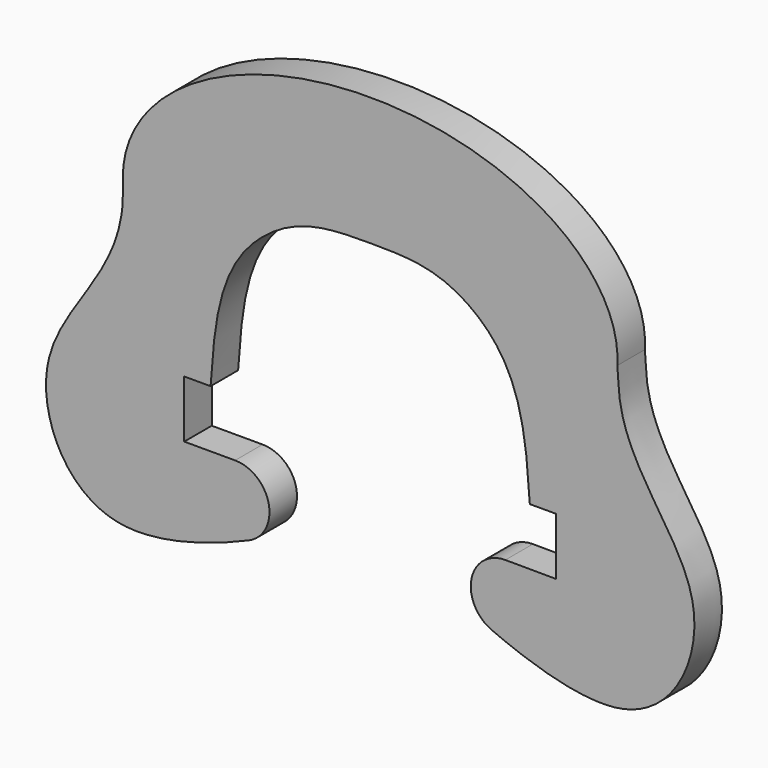
from build123d import *

# Parameters (mm, degrees)
F1_DEPTH = 3


# Not quite as in the source:
# - ends of sketch curves that miss each other by under 0.0002 mm in the source are joined
# - the dataset's text gives a spline's control points without its knots; the knots are read off the source's solid


with BuildPart() as f1:
    # F0 (on Front) → F1 (new body)
    with BuildSketch(Plane.XZ):
        with BuildLine():
            Line((-11.783002, -11.737941), (-16.216865, -11.737941))
            Line((-16.216865, -11.737941), (-16.216865, -6.737941))
            Line((-16.216865, -6.737941), (-13.918449, -6.737102))
            add(Edge.make_bspline(
                [(-13.918449, -6.737102), (-13.638513, -2.664171), (-13.2084, 3.593756), (-6.220813, 8.755675), (-2.060783, 8.765088), (-0.001865, 8.769746)],
                knots=[0, 0, 0, 0, 11.557339, 17.757478, 23.833112, 23.833112, 23.833112, 23.833112], degree=3))
            add(Edge.make_bspline(
                [(13.914719, -6.737102), (13.634783, -2.664171), (13.204671, 3.593756), (6.217084, 8.755675), (2.057054, 8.765088), (-0.001865, 8.769746)],
                knots=[0, 0, 0, 0, 11.557339, 17.757478, 23.833112, 23.833112, 23.833112, 23.833112], degree=3))
            Line((13.914719, -6.737102), (16.213135, -6.737941))
            Line((16.213135, -6.737941), (16.213135, -11.737941))
            Line((16.213135, -11.737941), (11.779312, -11.719301))
            ThreePointArc((11.779312, -11.719301), (8.8312342753, -14.1003719552), (10.5670700482, -17.4689818896))
            add(Edge.make_bspline(
                [(21.548331, 6.385136), (21.605514, 5.997937), (21.59991, -1.100257), (31.640163, -7.824719), (24.68515, -22.844764), (13.312431, -18.666716), (10.5670700482, -17.4689818896)],
                knots=[26.688985, 26.688985, 26.688985, 26.688985, 28.557776, 42.872008, 54.1154, 62.665306, 62.665306, 62.665306, 62.665306], degree=3))
            add(Edge.make_bspline(
                [(21.548331, 6.385136), (22.3407527768, 19.9695551789), (-0.001862111, 19.969557), (-22.3444769988, 19.9695588211), (-21.5520604233, 6.3851402115)],
                knots=[6.247711, 6.247711, 6.247711, 7.8539815, 7.8539815, 9.460252, 9.460252, 9.460252], degree=2, weights=[1, 0.6944541981, 1, 0.6944541981, 1]))
            add(Edge.make_bspline(
                [(-21.5520604233, 6.3851402115), (-21.534633, 6.02045), (-21.558871, -1.077705), (-31.627305, -7.759898), (-24.735498, -22.809049), (-13.345315, -18.678849), (-10.594943, -17.492667)],
                knots=[26.688985, 26.688985, 26.688985, 26.688985, 28.557776, 42.872008, 54.1154, 62.665306, 62.665306, 62.665306, 62.665306], degree=3))
            ThreePointArc((-10.594943, -17.492667), (-8.8449602866, -14.1313844153), (-11.783002, -11.737941))
        make_face()
    extrude(amount=F1_DEPTH)


solid = f1.part
